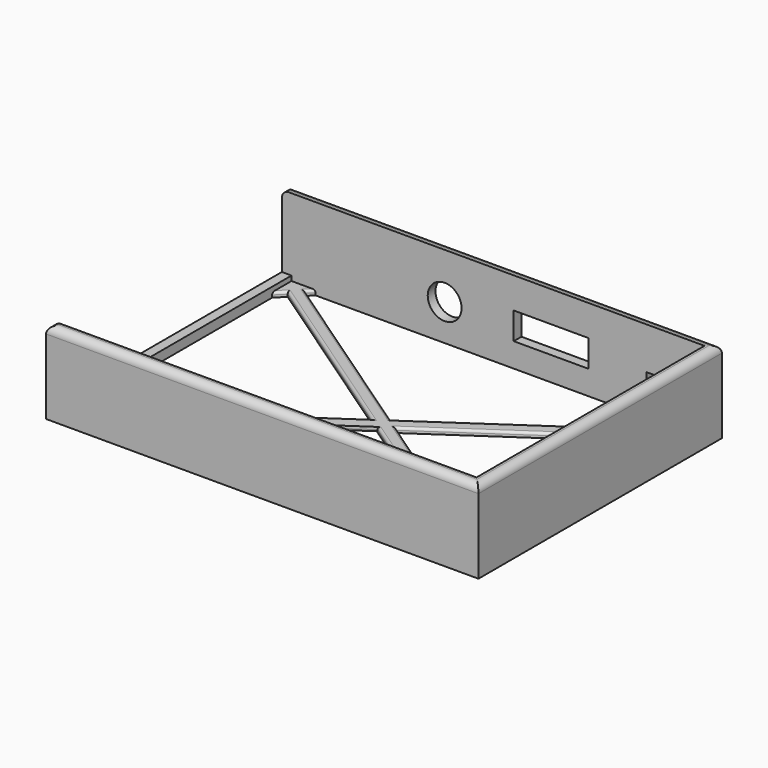
from build123d import *

# Parameters (mm, degrees)
F0_W     = 89.5
F0_H     = 63
F1_DEPTH = 17
F2_DEPTH = 1
F3_R     = 1.5
F4_R     = 0.49999
F5_W     = 7.7
F5_H     = 5
F5_W_2   = 15.5
F5_H_2   = 5.6
F5_R     = 3.5
F6_DEPTH = 25
F7_W     = 59
F7_H     = 13.5
F7_H_2   = 3.5
F8_DEPTH = 25


# Not quite as in the source:
# - a fillet or chamfer is up to 0.001 mm smaller than in the source, because OpenCascade refuses the exact size


with BuildPart() as f1:
    # F0 (on Top) → F1 (new body)
    with BuildSketch(Plane.XY):
        Rectangle(F0_W, F0_H)
        Polygon((-42.75, 24.5), (-42.75, 29.5), (-37.75, 29.5), (37.75, 29.5), (42.75, 29.5), (42.75, 24.5), (42.75, -24.5), (42.75, -29.5), (37.75, -29.5), (-37.75, -29.5), (-42.75, -29.5), (-42.75, -24.5), align=None, mode=Mode.SUBTRACT)
    extrude(amount=F1_DEPTH)

    # F0 (on Top) → F2 (join)
    with BuildSketch(Plane.XY):
        Polygon((-0.0146734692, 1.6726181109), (-38.9898385852, 28.2601614148), (-40.9670818505, 26.2829181495), (-2.4649122807, 0), (-40.9670818505, -26.2829181495), (-38.9670818505, -28.2829181495), (0, -1.6826347305), (38.9670818505, -28.2829181495), (40.96658534, -26.28341466), (2.4510848657, -0.0094390737), (40.9670818505, 26.2829181495), (38.9670818505, 28.2829181495), align=None)
        Polygon((-37.75, 29.5), (-42.75, 29.5), (-42.75, 24.5), (-40.9670818505, 26.2829181495), (-38.9898385852, 28.2601614148), align=None)
        Polygon((42.75, 29.5), (37.75, 29.5), (38.9670818505, 28.2829181495), (40.9670818505, 26.2829181495), (42.75, 24.5), align=None)
        Polygon((42.75, -29.5), (42.75, -24.5), (40.96658534, -26.28341466), (38.9670818505, -28.2829181495), (37.75, -29.5), align=None)
        Polygon((-40.9670818505, -26.2829181495), (-42.75, -24.5), (-42.75, -29.5), (-37.75, -29.5), (-38.9670818505, -28.2829181495), align=None)
    extrude(amount=F2_DEPTH)

    # F3
    f3_edges = [f1.edges().sort_by_distance(p)[0] for p in [
        (0, 31.5, 17),
        (-44.75, 0, 17),
        (0, -31.5, 17),
        (44.75, 0, 17),
    ]]
    fillet(f3_edges, radius=F3_R)

    # F4 (radius 0.5 in the source; OpenCascade refuses exactly that, so slightly less here)
    f4_edges = [f1.edges().sort_by_distance(p)[0] for p in [
        (-19.502256, 14.96639, 1),
        (-21.715997, 13.141459, 1),
        (19.476204, 14.977768, 1),
        (21.709083, 13.13674, 1),
        (-21.715997, -13.141459, 1),
        (-19.483541, -14.982776, 0),
        (19.483541, -14.982776, 1),
        (21.708835, -13.146427, 1),
        (-41.858541, 25.391459, 1),
        (-38.369919, 28.880081, 1),
        (41.858541, 25.391459, 1),
        (38.358541, 28.891459, 1),
        (-41.858541, -25.391459, 1),
        (-38.358541, -28.891459, 1),
        (41.858293, -25.391707, 1),
        (38.358541, -28.891459, 1),
    ]]
    fillet(f4_edges, radius=F4_R)

    # F5 (on face) → F6 (cut)
    with BuildSketch(Plane(origin=(0, 31.5, 0), x_dir=(-1, 0, 0), z_dir=(0, 1, 0))):
        with Locations((-34.6, 5.8)):
            Rectangle(F5_W, F5_H)
        with Locations((-11, 7.8)):
            Rectangle(F5_W_2, F5_H_2)
        with Locations((11.0494399613, 7.5)):
            Circle(F5_R)
    extrude(amount=-F6_DEPTH, mode=Mode.SUBTRACT)

    # F7 (on face) → F8 (cut)
    with BuildSketch(Plane(origin=(-44.75, 0, 0), x_dir=(0, -1, 0), z_dir=(-1, 0, 0))):
        with Locations((0, 8.75)):
            Rectangle(F7_W, F7_H)
        with Locations((0, 17.25)):
            Rectangle(F7_W, F7_H_2)
    extrude(amount=-F8_DEPTH, mode=Mode.SUBTRACT)


solid = f1.part
